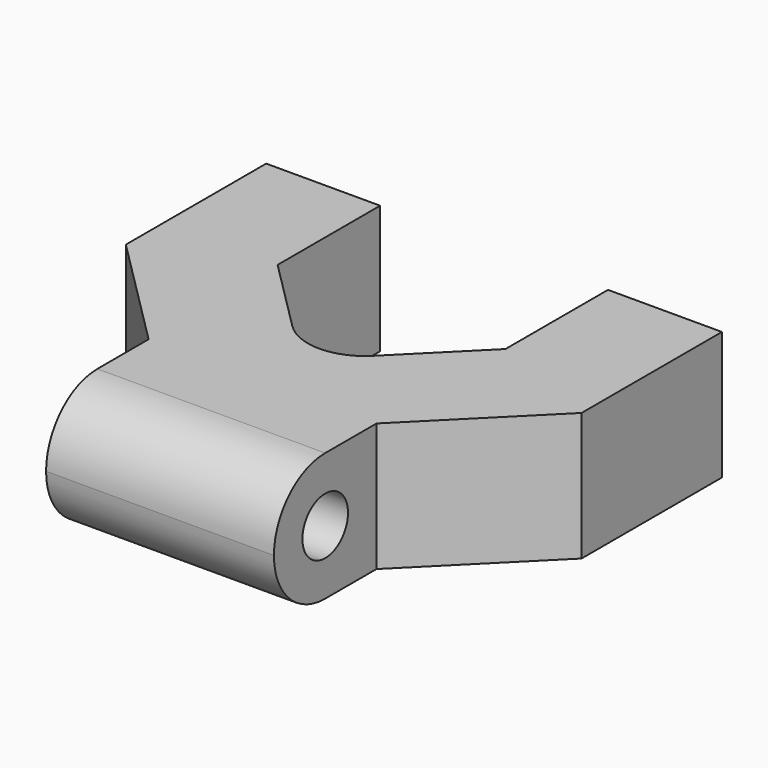
from build123d import *

# Parameters (mm, degrees)
F1_DEPTH = 4.5
F2_R     = 2
F4_R     = 1
F5_DEPTH = 25
F6_R     = 2.25
F7_R     = 2.24999


# Not quite as in the source:
# - a fillet or chamfer is up to 0.001 mm smaller than in the source, because OpenCascade refuses the exact size


with BuildPart() as f1:
    # F0 (on Top) → F1 (new body)
    with BuildSketch(Plane.XY):
        Polygon((12.6486692298, 5.0720985499), (12.6486692298, -1.0879014501), (16.6486692298, -1.0879014501), (16.6486692298, 3.4120985499), (20.6486692298, 7.4120985499), (20.6486692298, 13.5720985499), (16.6486692298, 13.5720985499), (16.6486692298, 9.0720985499), align=None)
        Polygon((8.6486692298, -1.0879014501), (12.6486692298, -1.0879014501), (12.6486692298, 5.0720985499), (8.6486692298, 9.0720985499), (8.6486692298, 13.5720985499), (4.6486692298, 13.5720985499), (4.6486692298, 7.4120985499), (8.6486692298, 3.4120985499), align=None)
    extrude(amount=F1_DEPTH)

    # F2
    f2_edges = [f1.edges().sort_by_distance(p)[0] for p in [
        (12.648669, 5.072099, 2.25),
    ]]
    fillet(f2_edges, radius=F2_R)

    # F4 (on face) → F5 (cut)
    with BuildSketch(Plane.YZ.offset(16.6486692298)):
        with Locations((1.1620985499, 2.25)):
            Circle(F4_R)
    extrude(amount=-F5_DEPTH, mode=Mode.SUBTRACT)

    # F6
    f6_edges = [f1.edges().sort_by_distance(p)[0] for p in [
        (12.648669, -1.087901, 0),
    ]]
    fillet(f6_edges, radius=F6_R)

    # F7 (radius 2.25 in the source; OpenCascade refuses exactly that, so slightly less here)
    f7_edges = [f1.edges().sort_by_distance(p)[0] for p in [
        (12.648669, -1.087901, 4.5),
    ]]
    fillet(f7_edges, radius=F7_R)


solid = f1.part
